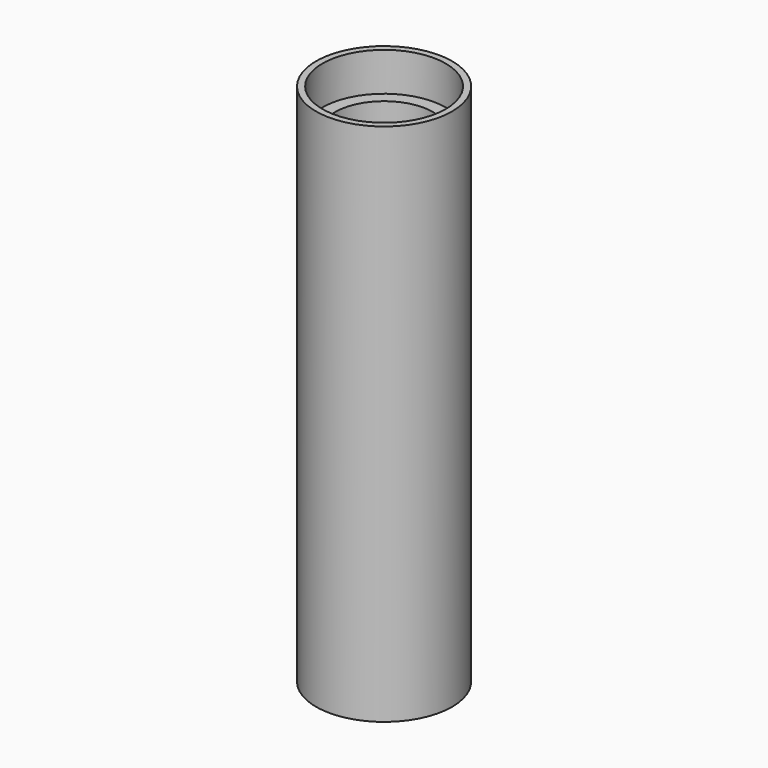
from build123d import *

# Parameters (mm, degrees)
F0_R        = 12.3317
F0_R_2      = 11.176
F1_DEPTH    = 47.5
F0_R_3      = 8.89
F2_DEPTH    = 40.5
F3_S5_R     = 11.176
F3_T6_DEPTH = 18


# Not quite as in the source:
# - a fillet or chamfer that OpenCascade refuses, or shapes differently, is made with other operations: its cross-section is extruded or revolved along the edge and cut away or added


with BuildPart() as f1:
    # F0 (on Top) → F1 (new body, symmetric)
    with BuildSketch(Plane.XY):
        Circle(F0_R)
        Circle(F0_R_2, mode=Mode.SUBTRACT)
    extrude(amount=F1_DEPTH, both=True)

    # F0 (on Top) → F2 (join, symmetric)
    with BuildSketch(Plane.XY):
        Circle(F0_R_2)
        Circle(F0_R_3, mode=Mode.SUBTRACT)
    extrude(amount=F2_DEPTH, both=True)

    # F3: chamfer of 2.54 on 1 edges, made by hand


with BuildPart() as f3_tool2:
    # F3_s3 → F3_t4 (revolve)
    with BuildSketch(Plane.XZ):
        Polygon((11.43, -40.5), (8.89, -37.96), (8.89, -40.5), align=None)
    revolve(axis=Axis((0, 0, -40.5), (0, 0, 1)))

    # F3_s5 → F3_t6 (intersect, symmetric)
    with BuildSketch(Plane.XY.offset(-39.2)):
        Circle(F3_S5_R)
    extrude(amount=F3_T6_DEPTH, both=True, mode=Mode.INTERSECT)


with BuildPart() as f1_1:
    add(f1.part)

    # F3_t1: cut F3_tool2
    add(f3_tool2.part, mode=Mode.SUBTRACT)


solid = f1_1.part
